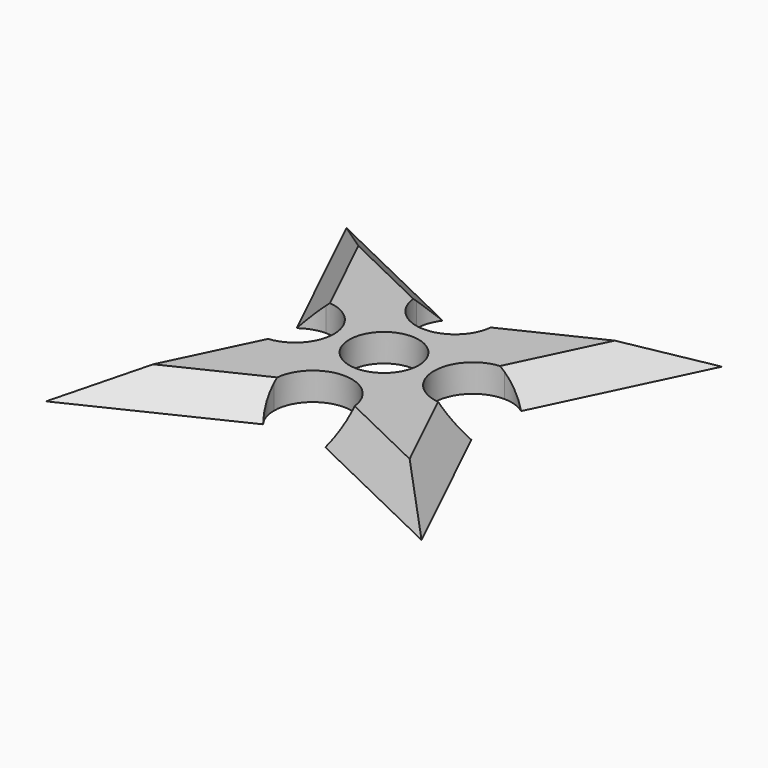
from build123d import *

# Parameters (mm, degrees)
F0_R     = 6.35
F1_DEPTH = 5.08
F2_SIZE  = 5.07999


# Not quite as in the source:
# - a fillet or chamfer is up to 0.001 mm smaller than in the source, because OpenCascade refuses the exact size


with BuildPart() as f1:
    # F0 (on Top) → F1 (new body)
    with BuildSketch(Plane.XY):
        with BuildLine():
            ThreePointArc((-16.2956875, 7.1118892639), (-12.5723585695, 12.5723585695), (-7.1118892639, 16.2956875))
            ThreePointArc((-7.1118892639, 16.2956875), (-6.7408857543, 18.5233780558), (-5.6901704054, 20.5224393535))
            Line((-5.6901704054, 20.5224393535), (-34.321730181, 34.321730181))
            Line((-34.321730181, 34.321730181), (-20.5224393535, 5.6901704054))
            ThreePointArc((-20.5224393535, 5.6901704054), (-18.5233780558, 6.7408857543), (-16.2956875, 7.1118892639))
        make_face()
        with BuildLine():
            ThreePointArc((16.2956875, -7.1118892639), (9.144, 0), (16.2956875, 7.1118892639))
            ThreePointArc((16.2956875, 7.1118892639), (12.5723585695, 12.5723585695), (7.1118892639, 16.2956875))
            ThreePointArc((7.1118892639, 16.2956875), (7.1119723159, 16.2758438272), (7.112, 16.256))
            ThreePointArc((7.112, 16.256), (-0.0198438272, 9.1440276841), (-7.1118892639, 16.2956875))
            ThreePointArc((-7.1118892639, 16.2956875), (-12.5723585695, 12.5723585695), (-16.2956875, 7.1118892639))
            ThreePointArc((-16.2956875, 7.1118892639), (-11.2411078526, 5.042955557), (-9.144, 0))
            ThreePointArc((-9.144, 0), (-11.2411078526, -5.042955557), (-16.2956875, -7.1118892639))
            ThreePointArc((-16.2956875, -7.1118892639), (-12.5723585695, -12.5723585695), (-7.1118892639, -16.2956875))
            ThreePointArc((-7.1118892639, -16.2956875), (-0.0198438272, -9.1440276841), (7.112, -16.256))
            ThreePointArc((7.112, -16.256), (7.1119723159, -16.2758438272), (7.1118892639, -16.2956875))
            ThreePointArc((7.1118892639, -16.2956875), (12.5723585695, -12.5723585695), (16.2956875, -7.1118892639))
        make_face()
        Circle(F0_R, mode=Mode.SUBTRACT)
        with BuildLine():
            ThreePointArc((7.1118892639, 16.2956875), (12.5723585695, 12.5723585695), (16.2956875, 7.1118892639))
            ThreePointArc((16.2956875, 7.1118892639), (18.5233780558, 6.7408857543), (20.5224393535, 5.6901704054))
            Line((20.5224393535, 5.6901704054), (34.321730181, 34.321730181))
            Line((34.321730181, 34.321730181), (5.6901704054, 20.5224393535))
            ThreePointArc((5.6901704054, 20.5224393535), (6.7408857543, 18.5233780558), (7.1118892639, 16.2956875))
        make_face()
        with BuildLine():
            ThreePointArc((20.5224393535, -5.6901704054), (18.5233780558, -6.7408857543), (16.2956875, -7.1118892639))
            ThreePointArc((16.2956875, -7.1118892639), (12.5723585695, -12.5723585695), (7.1118892639, -16.2956875))
            ThreePointArc((7.1118892639, -16.2956875), (6.7408857543, -18.5233780558), (5.6901704054, -20.5224393535))
            Line((5.6901704054, -20.5224393535), (34.321730181, -34.321730181))
            Line((34.321730181, -34.321730181), (20.5224393535, -5.6901704054))
        make_face()
        with BuildLine():
            ThreePointArc((-5.6901704054, -20.5224393535), (-6.7408857543, -18.5233780558), (-7.1118892639, -16.2956875))
            ThreePointArc((-7.1118892639, -16.2956875), (-12.5723585695, -12.5723585695), (-16.2956875, -7.1118892639))
            ThreePointArc((-16.2956875, -7.1118892639), (-18.5233780558, -6.7408857543), (-20.5224393535, -5.6901704054))
            Line((-20.5224393535, -5.6901704054), (-34.321730181, -34.321730181))
            Line((-34.321730181, -34.321730181), (-5.6901704054, -20.5224393535))
        make_face()
    extrude(amount=F1_DEPTH)

    # F2 (size 5.08 in the source; OpenCascade refuses exactly that, so slightly less here)
    f2_edges = [f1.edges().sort_by_distance(p)[0] for p in [
        (-27.422085, 20.00595, 5.08),
        (-20.00595, 27.422085, 5.08),
        (20.00595, 27.422085, 5.08),
        (27.422085, 20.00595, 5.08),
        (27.422085, -20.00595, 5.08),
        (20.00595, -27.422085, 5.08),
        (-20.00595, -27.422085, 5.08),
        (-27.422085, -20.00595, 5.08),
    ]]
    chamfer(f2_edges, length=F2_SIZE)


solid = f1.part
